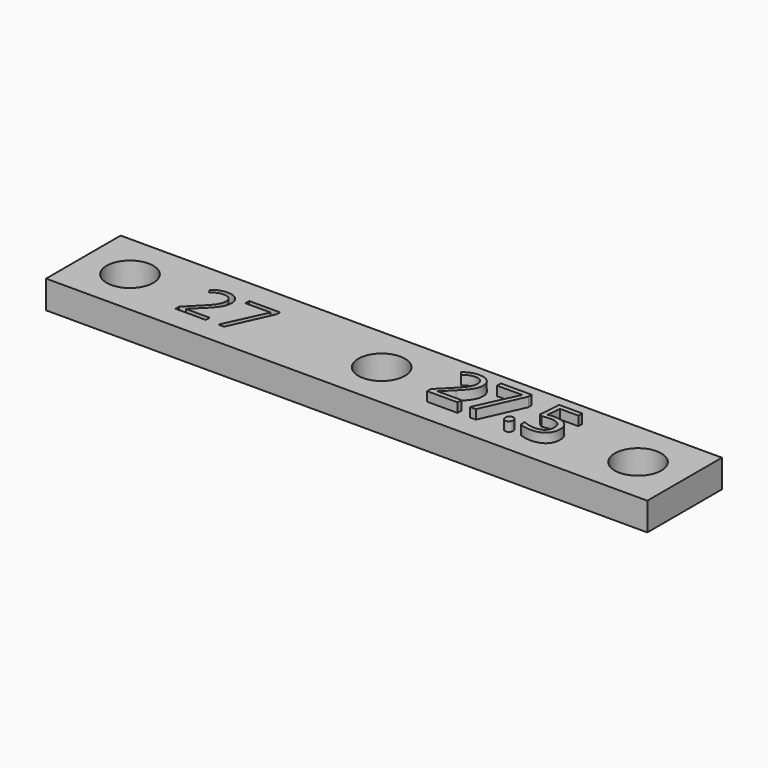
from build123d import *

# Parameters (mm, degrees)
F0_R         = 2.5
F1_DEPTH     = 3
F0_TEXT_SIZE = 6.9444444444
F2_DEPTH     = 4


# Not quite as in the source:
# - Text() gives the source's letters only with a copy of the font that has no kerning and outlines rounded to 1/6400 em; it was checked with that copy


with BuildPart() as f1:
    # F0 (on Top) → F1 (new body)
    with BuildSketch(Plane.XY):
        Polygon((-32, 5), (-32, 0), (-32, -5), (32.5, -5), (32.5, 0), (32.5, 5), align=None)
        Polygon((-14.9006706819, -2.5), (-15.5245856125, -2.5), (-13.4705491541, 1.9390190972), (-16.1723720708, 1.9390190972), (-16.1723720708, 2.4576822917), (-12.8737609597, 2.4576822917), (-12.8737609597, 2.0062934028), align=None, mode=Mode.SUBTRACT)
        with BuildLine():
            add(Edge.make_bspline(
                [(15.1076843528, -2.4918619792), (14.9942945959, -2.3849826389), (14.9942945959, -2.1408420139)],
                knots=[0, 0, 0, 1, 1, 1], degree=2))
            add(Edge.make_bspline(
                [(14.9942945959, -2.1408420139), (14.9942945959, -1.9129774306), (15.0979187278, -1.7963324653)],
                knots=[0, 0, 0, 1, 1, 1], degree=2))
            add(Edge.make_bspline(
                [(15.0979187278, -1.7963324653), (15.2015428598, -1.6796875), (15.3946852209, -1.6796875)],
                knots=[0, 0, 0, 1, 1, 1], degree=2))
            add(Edge.make_bspline(
                [(15.3946852209, -1.6796875), (15.5910827903, -1.6796875), (15.7012173389, -1.7963324653)],
                knots=[0, 0, 0, 1, 1, 1], degree=2))
            add(Edge.make_bspline(
                [(15.7012173389, -1.7963324653), (15.8113518875, -1.9129774306), (15.8113518875, -2.1408420139)],
                knots=[0, 0, 0, 1, 1, 1], degree=2))
            add(Edge.make_bspline(
                [(15.8113518875, -2.1408420139), (15.8113518875, -2.3611111111), (15.6995897348, -2.4799262153)],
                knots=[0, 0, 0, 1, 1, 1], degree=2))
            add(Edge.make_bspline(
                [(15.6995897348, -2.4799262153), (15.587827582, -2.5987413194), (15.3946852209, -2.5987413194)],
                knots=[0, 0, 0, 1, 1, 1], degree=2))
            add(Edge.make_bspline(
                [(15.3946852209, -2.5987413194), (15.2210741098, -2.5987413194), (15.1076843528, -2.4918619792)],
                knots=[0, 0, 0, 1, 1, 1], degree=2))
        make_face(mode=Mode.SUBTRACT)
        Polygon((12.0993293181, -2.5), (11.4754143875, -2.5), (13.5294508459, 1.9390190972), (10.8276279292, 1.9390190972), (10.8276279292, 2.4576822917), (14.1262390403, 2.4576822917), (14.1262390403, 2.0062934028), align=None, mode=Mode.SUBTRACT)
        with BuildLine():
            add(Edge.make_bspline(
                [(17.4389560542, 0.4503038194), (17.8284959848, 0.5284288194), (18.2158657764, 0.5284288194)],
                knots=[0, 0, 0, 1, 1, 1], degree=2))
            add(Edge.make_bspline(
                [(18.2158657764, 0.5284288194), (18.9992859153, 0.5284288194), (19.4485046653, 0.1399739583)],
                knots=[0, 0, 0, 1, 1, 1], degree=2))
            add(Edge.make_bspline(
                [(19.4485046653, 0.1399739583), (19.8977234153, -0.2484809028), (19.8977234153, -0.9233940972)],
                knots=[0, 0, 0, 1, 1, 1], degree=2))
            add(Edge.make_bspline(
                [(19.8977234153, -0.9233940972), (19.8977234153, -1.6927083333), (19.4078145611, -2.1305338542)],
                knots=[0, 0, 0, 1, 1, 1], degree=2))
            add(Edge.make_bspline(
                [(19.4078145611, -2.1305338542), (18.917905707, -2.568359375), (18.0563605681, -2.568359375)],
                knots=[0, 0, 0, 1, 1, 1], degree=2))
            add(Edge.make_bspline(
                [(18.0563605681, -2.568359375), (17.218686957, -2.568359375), (16.7781487625, -2.3003472222)],
                knots=[0, 0, 0, 1, 1, 1], degree=2))
            Line((16.7781487625, -2.3003472222), (16.7781487625, -1.7578125))
            add(Edge.make_bspline(
                [(16.7781487625, -1.7578125), (17.0146939014, -1.9097222222), (17.3673414709, -1.9965277778)],
                knots=[0, 0, 0, 1, 1, 1], degree=2))
            add(Edge.make_bspline(
                [(17.3673414709, -1.9965277778), (17.7199890403, -2.0833333333), (18.0628709848, -2.0833333333)],
                knots=[0, 0, 0, 1, 1, 1], degree=2))
            add(Edge.make_bspline(
                [(18.0628709848, -2.0833333333), (18.6596591792, -2.0833333333), (18.990062825, -1.8017578125)],
                knots=[0, 0, 0, 1, 1, 1], degree=2))
            add(Edge.make_bspline(
                [(18.990062825, -1.8017578125), (19.3204664709, -1.5201822917), (19.3204664709, -0.9874131944)],
                knots=[0, 0, 0, 1, 1, 1], degree=2))
            add(Edge.make_bspline(
                [(19.3204664709, -0.9874131944), (19.3204664709, 0.0499131944), (18.0498501514, 0.0499131944)],
                knots=[0, 0, 0, 1, 1, 1], degree=2))
            add(Edge.make_bspline(
                [(18.0498501514, 0.0499131944), (17.7275845264, 0.0499131944), (17.1883050125, -0.048828125)],
                knots=[0, 0, 0, 1, 1, 1], degree=2))
            Line((17.1883050125, -0.048828125), (16.896421332, 0.1378038194))
            Line((16.896421332, 0.1378038194), (17.0830532764, 2.4576822917))
            Line((17.0830532764, 2.4576822917), (19.5483310542, 2.4576822917))
            Line((19.5483310542, 2.4576822917), (19.5483310542, 1.9390190972))
            Line((19.5483310542, 1.9390190972), (17.5648241098, 1.9390190972))
            Line((17.5648241098, 1.9390190972), (17.4389560542, 0.4503038194))
        make_face(mode=Mode.SUBTRACT)
        with Locations((-27, 0)):
            Circle(F0_R, mode=Mode.SUBTRACT)
        with BuildLine():
            Line((-16.8635613069, -1.9780815972), (-16.8635613069, -2.5))
            Line((-16.8635613069, -2.5), (-20.1220248486, -2.5))
            Line((-20.1220248486, -2.5), (-20.1220248486, -2.0149739583))
            Line((-20.1220248486, -2.0149739583), (-18.8166863069, -0.703125))
            add(Edge.make_bspline(
                [(-18.8166863069, -0.703125), (-18.2198981125, -0.0987413194), (-18.0300109597, 0.1589626736)],
                knots=[0, 0, 0, 1, 1, 1], degree=2))
            add(Edge.make_bspline(
                [(-18.0300109597, 0.1589626736), (-17.8401238069, 0.4166666667), (-17.7451802305, 0.6608072917)],
                knots=[0, 0, 0, 1, 1, 1], degree=2))
            add(Edge.make_bspline(
                [(-17.7451802305, 0.6608072917), (-17.6502366541, 0.9049479167), (-17.6502366541, 1.1859809028)],
                knots=[0, 0, 0, 1, 1, 1], degree=2))
            add(Edge.make_bspline(
                [(-17.6502366541, 1.1859809028), (-17.6502366541, 1.5831163194), (-17.8911220708, 1.8153211806)],
                knots=[0, 0, 0, 1, 1, 1], degree=2))
            add(Edge.make_bspline(
                [(-17.8911220708, 1.8153211806), (-18.1320074875, 2.0475260417), (-18.5595248486, 2.0475260417)],
                knots=[0, 0, 0, 1, 1, 1], degree=2))
            add(Edge.make_bspline(
                [(-18.5595248486, 2.0475260417), (-18.8676845708, 2.0475260417), (-19.1443772791, 1.9455295139)],
                knots=[0, 0, 0, 1, 1, 1], degree=2))
            add(Edge.make_bspline(
                [(-19.1443772791, 1.9455295139), (-19.4210699875, 1.8435329861), (-19.7596116541, 1.5755208333)],
                knots=[0, 0, 0, 1, 1, 1], degree=2))
            Line((-19.7596116541, 1.5755208333), (-20.0580057514, 1.9585503472))
            add(Edge.make_bspline(
                [(-20.0580057514, 1.9585503472), (-19.3733269319, 2.5282118056), (-18.5660352652, 2.5282118056)],
                knots=[0, 0, 0, 1, 1, 1], degree=2))
            add(Edge.make_bspline(
                [(-18.5660352652, 2.5282118056), (-17.867250543, 2.5282118056), (-17.4706576611, 2.1706814236)],
                knots=[0, 0, 0, 1, 1, 1], degree=2))
            add(Edge.make_bspline(
                [(-17.4706576611, 2.1706814236), (-17.0740647791, 1.8131510417), (-17.0740647791, 1.2098524306)],
                knots=[0, 0, 0, 1, 1, 1], degree=2))
            add(Edge.make_bspline(
                [(-17.0740647791, 1.2098524306), (-17.0740647791, 0.7378472222), (-17.3388217236, 0.2766927083)],
                knots=[0, 0, 0, 1, 1, 1], degree=2))
            add(Edge.make_bspline(
                [(-17.3388217236, 0.2766927083), (-17.603578668, -0.1844618056), (-18.3284050569, -0.8897569444)],
                knots=[0, 0, 0, 1, 1, 1], degree=2))
            Line((-18.3284050569, -0.8897569444), (-19.4134745014, -1.9509548611))
            Line((-19.4134745014, -1.9509548611), (-19.4134745014, -1.9780815972))
            Line((-19.4134745014, -1.9780815972), (-16.8635613069, -1.9780815972))
        make_face(mode=Mode.SUBTRACT)
        Circle(F0_R, mode=Mode.SUBTRACT)
        with BuildLine():
            Line((10.1364386931, -1.9780815972), (10.1364386931, -2.5))
            Line((10.1364386931, -2.5), (6.8779751514, -2.5))
            Line((6.8779751514, -2.5), (6.8779751514, -2.0149739583))
            Line((6.8779751514, -2.0149739583), (8.1833136931, -0.703125))
            add(Edge.make_bspline(
                [(8.1833136931, -0.703125), (8.7801018875, -0.0987413194), (8.9699890403, 0.1589626736)],
                knots=[0, 0, 0, 1, 1, 1], degree=2))
            add(Edge.make_bspline(
                [(8.9699890403, 0.1589626736), (9.1598761931, 0.4166666667), (9.2548197695, 0.6608072917)],
                knots=[0, 0, 0, 1, 1, 1], degree=2))
            add(Edge.make_bspline(
                [(9.2548197695, 0.6608072917), (9.3497633459, 0.9049479167), (9.3497633459, 1.1859809028)],
                knots=[0, 0, 0, 1, 1, 1], degree=2))
            add(Edge.make_bspline(
                [(9.3497633459, 1.1859809028), (9.3497633459, 1.5831163194), (9.1088779292, 1.8153211806)],
                knots=[0, 0, 0, 1, 1, 1], degree=2))
            add(Edge.make_bspline(
                [(9.1088779292, 1.8153211806), (8.8679925125, 2.0475260417), (8.4404751514, 2.0475260417)],
                knots=[0, 0, 0, 1, 1, 1], degree=2))
            add(Edge.make_bspline(
                [(8.4404751514, 2.0475260417), (8.1323154292, 2.0475260417), (7.8556227209, 1.9455295139)],
                knots=[0, 0, 0, 1, 1, 1], degree=2))
            add(Edge.make_bspline(
                [(7.8556227209, 1.9455295139), (7.5789300125, 1.8435329861), (7.2403883459, 1.5755208333)],
                knots=[0, 0, 0, 1, 1, 1], degree=2))
            Line((7.2403883459, 1.5755208333), (6.9419942486, 1.9585503472))
            add(Edge.make_bspline(
                [(6.9419942486, 1.9585503472), (7.6266730681, 2.5282118056), (8.4339647348, 2.5282118056)],
                knots=[0, 0, 0, 1, 1, 1], degree=2))
            add(Edge.make_bspline(
                [(8.4339647348, 2.5282118056), (9.132749457, 2.5282118056), (9.5293423389, 2.1706814236)],
                knots=[0, 0, 0, 1, 1, 1], degree=2))
            add(Edge.make_bspline(
                [(9.5293423389, 2.1706814236), (9.9259352209, 1.8131510417), (9.9259352209, 1.2098524306)],
                knots=[0, 0, 0, 1, 1, 1], degree=2))
            add(Edge.make_bspline(
                [(9.9259352209, 1.2098524306), (9.9259352209, 0.7378472222), (9.6611782764, 0.2766927083)],
                knots=[0, 0, 0, 1, 1, 1], degree=2))
            add(Edge.make_bspline(
                [(9.6611782764, 0.2766927083), (9.396421332, -0.1844618056), (8.6715949431, -0.8897569444)],
                knots=[0, 0, 0, 1, 1, 1], degree=2))
            Line((8.6715949431, -0.8897569444), (7.5865254986, -1.9509548611))
            Line((7.5865254986, -1.9509548611), (7.5865254986, -1.9780815972))
            Line((7.5865254986, -1.9780815972), (10.1364386931, -1.9780815972))
        make_face(mode=Mode.SUBTRACT)
        with Locations((27.5, 0)):
            Circle(F0_R, mode=Mode.SUBTRACT)
    extrude(amount=F1_DEPTH)

    # F0 (on Top) → F2 (join)
    with BuildSketch(Plane.XY):
        with Locations((6.5383484153, -2.5)):
            Text('27.5', F0_TEXT_SIZE, font='Open Sans', text_align=(TextAlign.LEFT, TextAlign.BOTTOM))
    extrude(amount=F2_DEPTH)


solid = f1.part
